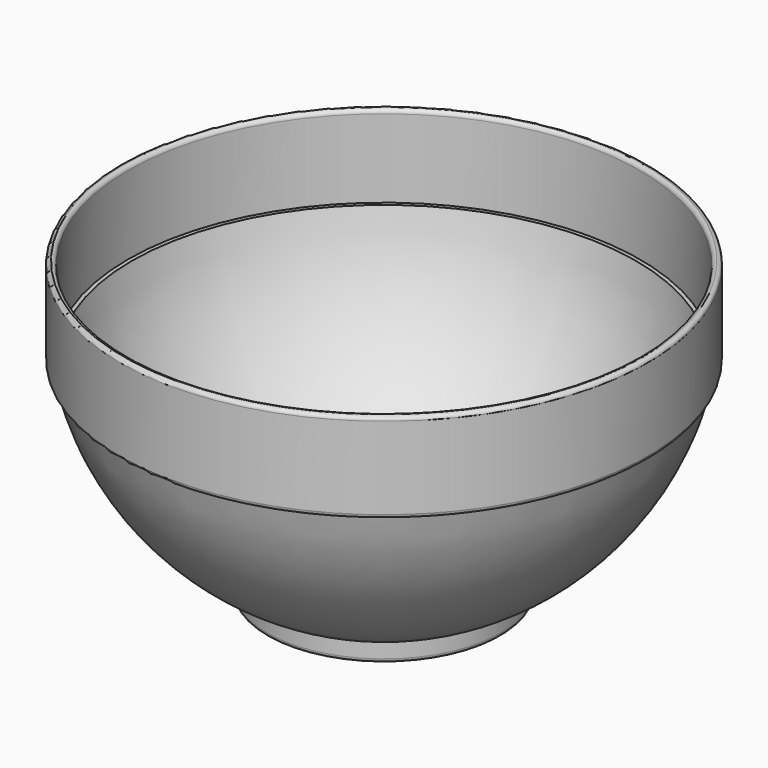
from build123d import *

# Parameters (mm, degrees)
F2_R = 0.99999


# Not quite as in the source:
# - a fillet or chamfer is up to 0.001 mm smaller than in the source, because OpenCascade refuses the exact size


with BuildPart() as f1:
    # F0 (on Front) → F1 (revolve)
    with BuildSketch(Plane.XZ):
        with BuildLine():
            Line((-64.5, 52), (-65.5, 52))
            Line((-65.5, 52), (-65.5, 73))
            Line((-65.5, 73), (-67.5, 73))
            Line((-67.5, 73), (-67.5, 50))
            Line((-67.5, 50), (-66.1449700482, 50))
            ThreePointArc((-66.1449700482, 50), (-53.4398255255, 22.2737739938), (-30, 2.761242502))
            Line((-30, 2.761242502), (-30, -2))
            Line((-30, -2), (0, -2))
            Line((0, -2), (0, 0))
            Line((0, 0), (-28, 0))
            Line((-28, 0), (-28, 4))
            ThreePointArc((-28, 4), (-51.9728387009, 23.6482580712), (-64.5, 52))
        make_face()
    revolve(axis=Axis((0, 0, -1), (0, 0, -1)))

    # F2 (radius 1 in the source; OpenCascade refuses exactly that, so slightly less here)
    f2_edges = [f1.edges().sort_by_distance(p)[0] for p in [
        (67.5, 0, 73),
        (65.5, 0, 73),
        (67.5, 0, 50),
        (30, 0, -2),
    ]]
    fillet(f2_edges, radius=F2_R)


solid = f1.part
